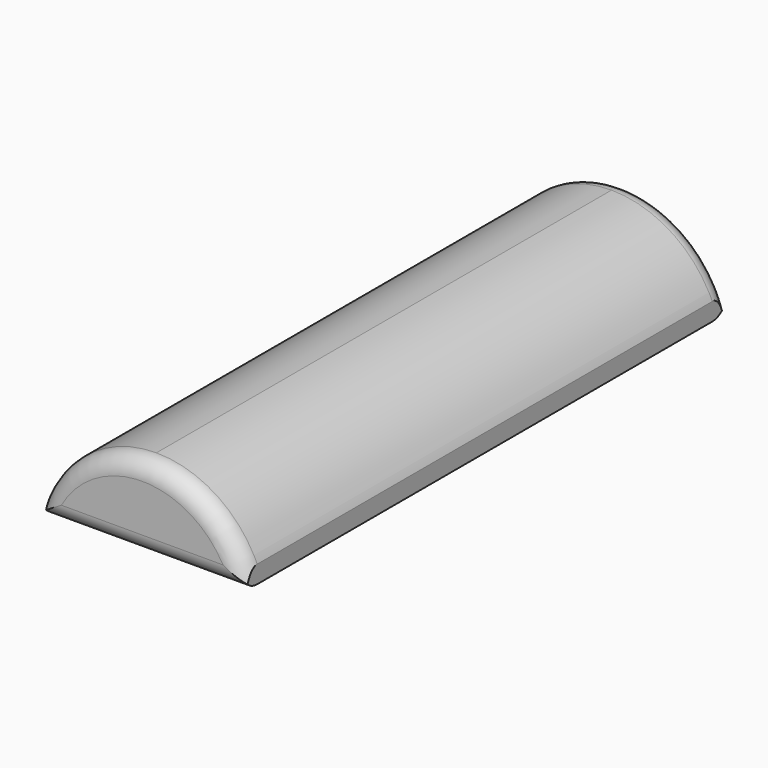
from build123d import *

# Parameters (mm, degrees)
F0_W        = 17
F0_H        = 3
F1_DEPTH    = 102
F2_T2_ANGLE = 177.7767208829
F2_T4_ANGLE = 177.7767208829
F2_T5_DEPTH = 44.8663690461
F2_T7_DEPTH = 44.8663690461


# Not quite as in the source:
# - a fillet or chamfer that OpenCascade refuses, or shapes differently, is made with other operations: its cross-section is extruded or revolved along the edge and cut away or added


with BuildPart() as f1:
    # F0 (on Front) → F1 (new body)
    with BuildSketch(Plane.XZ):
        with BuildLine():
            ThreePointArc((0, 7), (-10.1242283657, 4.0101711106), (-17, -4))
            Line((-17, -4), (0, -4))
            Line((0, -4), (0, 0))
            Line((0, 0), (0, 7))
        make_face()
        with BuildLine():
            Line((0, 0), (0, -4))
            Line((0, -4), (17, -4))
            ThreePointArc((17, -4), (10.1242283657, 4.0101711106), (0, 7))
            Line((0, 7), (0, 0))
        make_face()
        with Locations((-8.5, -5.5)):
            Rectangle(F0_W, F0_H)
        with Locations((8.5, -5.5)):
            Rectangle(F0_W, F0_H)
    extrude(amount=F1_DEPTH)

    # F2: fillet of radius 3 on 8 edges, made by hand

    # F2_s1 → F2_t2 (revolve, cut)
    with BuildSketch(Plane(origin=(0.2257094032, 0, -11.6319839248), x_dir=(0, 1, 0), z_dir=(0.0194005532, 0, -0.9998117916))):
        with BuildLine():
            ThreePointArc((-3, 18.4106117448), (-0.8786796564, 17.5319320883), (0, 15.4106117448))
            Line((0, 15.4106117448), (0.06, 15.4106117448))
            Line((0.06, 15.4106117448), (0.06, 18.4706117448))
            Line((0.06, 18.4706117448), (-3, 18.4706117448))
            Line((-3, 18.4706117448), (-3, 18.4106117448))
        make_face()
    revolve(axis=Axis((0, 0, -11.6363636364), (0, -1, 0)), revolution_arc=F2_T2_ANGLE, mode=Mode.SUBTRACT)

    # F2_s3 → F2_t4 (revolve, cut)
    with BuildSketch(Plane(origin=(0.2257094032, 0, -11.6319839248), x_dir=(0, 1, 0), z_dir=(0.0194005532, 0, -0.9998117916))):
        with BuildLine():
            ThreePointArc((-99, 18.4106117448), (-101.1213203436, 17.5319320883), (-102, 15.4106117448))
            Line((-102, 15.4106117448), (-102.06, 15.4106117448))
            Line((-102.06, 15.4106117448), (-102.06, 18.4706117448))
            Line((-102.06, 18.4706117448), (-99, 18.4706117448))
            Line((-99, 18.4706117448), (-99, 18.4106117448))
        make_face()
    revolve(axis=Axis((0, -102, -11.6363636364), (0, -1, 0)), revolution_arc=F2_T4_ANGLE, mode=Mode.SUBTRACT)

    # F2_s6 → F2_t5 (cut)
    with BuildSketch(Plane.YZ.offset(-22.4331845231)):
        with BuildLine():
            ThreePointArc((-3, -7), (-0.8786796564, -6.1213203436), (0, -4))
            Line((0, -4), (0.06, -4))
            Line((0.06, -4), (0.06, -7.06))
            Line((0.06, -7.06), (-3, -7.06))
            Line((-3, -7.06), (-3, -7))
        make_face()
    extrude(amount=F2_T5_DEPTH, mode=Mode.SUBTRACT)

    # F2_s8 → F2_t7 (cut)
    with BuildSketch(Plane.YZ.offset(-22.4331845231)):
        with BuildLine():
            ThreePointArc((-99, -7), (-101.1213203436, -6.1213203436), (-102, -4))
            Line((-102, -4), (-102.06, -4))
            Line((-102.06, -4), (-102.06, -7.06))
            Line((-102.06, -7.06), (-99, -7.06))
            Line((-99, -7.06), (-99, -7))
        make_face()
    extrude(amount=F2_T7_DEPTH, mode=Mode.SUBTRACT)


solid = f1.part
